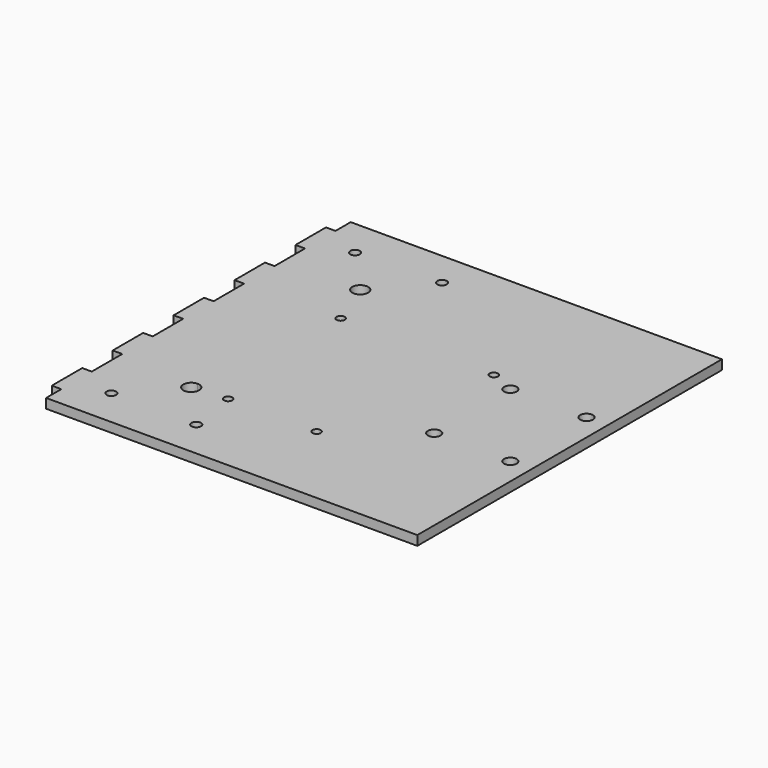
from build123d import *

# Parameters (mm, degrees)
F0_R     = 1.5
F0_R_2   = 2
F0_R_3   = 2.5
F1_DEPTH = 3


with BuildPart() as f1:
    # F0 (on Top) → F1 (new body)
    with BuildSketch(Plane.XY):
        Polygon((74.5058632415, 0), (74.5058632415, 60), (-42.4941367585, 60), (-42.4941367585, 54), (-45.4941367585, 54), (-45.4941367585, 42), (-42.4941367585, 42), (-42.4941367585, 30), (-45.4941367585, 30), (-45.4941367585, 18), (-42.4941367585, 18), (-42.4941367585, 6), (-45.4941367585, 6), (-45.4941367585, -6), (-42.4941367585, -6), (-42.4941367585, -17.9991139914), (-45.4941367585, -17.9991139914), (-45.4941367585, -29.9991139914), (-42.4941367585, -29.9991139914), (-42.4941367585, -42), (-45.4941367585, -42), (-45.4941367585, -54), (-42.4941367585, -54), (-42.4941367585, -60), (74.5058632415, -60), align=None)
        with Locations((-31.4941367585, -48)):
            Circle(F0_R, mode=Mode.SUBTRACT)
        with BuildLine():
            ThreePointArc((-15.6229661617, -33.2851748408), (-16.3557725378, -35.053514937), (-18.1245875184, -35.785174315))
            ThreePointArc((-18.1245875184, -35.785174315), (-20.6229656359, -33.2835534841), (-18.1213448049, -30.7851753666))
            ThreePointArc((-18.1213448049, -30.7851753666), (-16.3546260654, -31.517981217), (-15.6229661617, -33.2851748408))
        make_face(mode=Mode.SUBTRACT)
        with BuildLine():
            ThreePointArc((-3.2708819532, -48), (-4.7708819532, -49.5), (-6.2708819532, -48))
            ThreePointArc((-6.2708819532, -48), (-4.7708819532, -46.5), (-3.2708819532, -48))
        make_face(mode=Mode.SUBTRACT)
        with BuildLine():
            Line((35.8920598827, 17.1), (35.8920598827, 0))
            Line((35.8920598827, 0), (35.8920598827, -32.4))
            Line((35.8920598827, -32.4), (21.9920598827, -32.4))
            ThreePointArc((21.9920598827, -32.4), (20.6920598827, -33.7), (19.3920598827, -32.4))
            Line((19.3920598827, -32.4), (-5.9079401173, -32.4))
            ThreePointArc((-5.9079401173, -32.4), (-7.2079401173, -33.7), (-8.5079401173, -32.4))
            Line((-8.5079401173, -32.4), (-12.4079401173, -32.4))
            Line((-12.4079401173, -32.4), (-12.4079401173, 17.1))
            ThreePointArc((-12.4079401173, 17.1), (-13.3271789328, 19.3192388155), (-11.1079401173, 18.4))
            Line((-11.1079401173, 18.4), (34.5920598827, 18.4))
            ThreePointArc((34.5920598827, 18.4), (35.8920598827, 19.7), (37.1920598827, 18.4))
            ThreePointArc((37.1920598827, 18.4), (36.8112986983, 17.4807611845), (35.8920598827, 17.1))
        make_face(mode=Mode.SUBTRACT)
        with Locations((43.8302124143, -15)):
            Circle(F0_R_2, mode=Mode.SUBTRACT)
        with Locations((67.8302124143, -15)):
            Circle(F0_R_2, mode=Mode.SUBTRACT)
        with Locations((-18.1229661617, 33.2851748408)):
            Circle(F0_R_3, mode=Mode.SUBTRACT)
        with Locations((-31.4937761504, 48)):
            Circle(F0_R, mode=Mode.SUBTRACT)
        with Locations((-4.7708819532, 48.8354042139)):
            Circle(F0_R, mode=Mode.SUBTRACT)
        with Locations((43.8302124143, 15)):
            Circle(F0_R_2, mode=Mode.SUBTRACT)
        with Locations((67.8302124143, 15)):
            Circle(F0_R_2, mode=Mode.SUBTRACT)
        with BuildLine():
            Line((35.8920598827, -32.4), (35.8920598827, 0))
            Line((35.8920598827, 0), (35.8920598827, 17.1))
            ThreePointArc((35.8920598827, 17.1), (34.9728210672, 17.4807611845), (34.5920598827, 18.4))
            Line((34.5920598827, 18.4), (-11.1079401173, 18.4))
            ThreePointArc((-11.1079401173, 18.4), (-11.4887013017, 17.4807611845), (-12.4079401173, 17.1))
            Line((-12.4079401173, 17.1), (-12.4079401173, -32.4))
            Line((-12.4079401173, -32.4), (-8.5079401173, -32.4))
            ThreePointArc((-8.5079401173, -32.4), (-7.2079401173, -31.1), (-5.9079401173, -32.4))
            Line((-5.9079401173, -32.4), (19.3920598827, -32.4))
            ThreePointArc((19.3920598827, -32.4), (20.6920598827, -31.1), (21.9920598827, -32.4))
            Line((21.9920598827, -32.4), (35.8920598827, -32.4))
        make_face()
    extrude(amount=F1_DEPTH)


solid = f1.part
